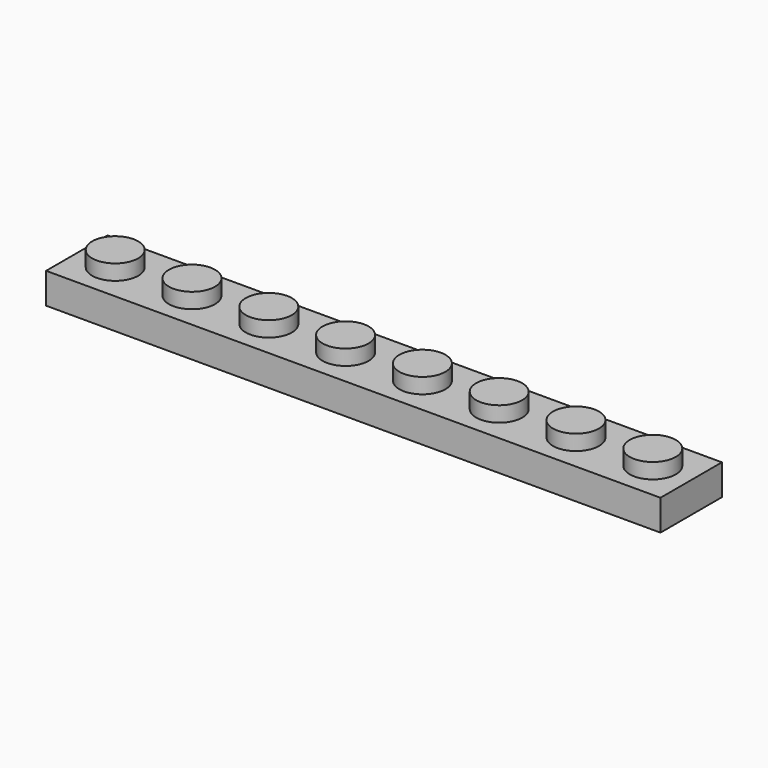
from build123d import *

# Parameters (mm, degrees)
F0_W     = 63.5
F0_H     = 7.9375
F0_R     = 2.38125
F1_DEPTH = 3.175
F2_DEPTH = 4.7625
F3_T     = -1.5875
F4_R     = 1.5875
F4_R_2   = 0.79375
F5_DEPTH = 1.5875


# Not quite as in the source:
# - a feature names something its author has since deleted; it is built from what else it names


with BuildPart() as f1:
    # F0 (on Top) → F1 (new body)
    with BuildSketch(Plane.XY):
        Rectangle(F0_W, F0_H)
        with Locations((-27.78125, 0)):
            Circle(F0_R, mode=Mode.SUBTRACT)
        with Locations((-19.84375, 0)):
            Circle(F0_R, mode=Mode.SUBTRACT)
        with Locations((-11.90625, 0)):
            Circle(F0_R, mode=Mode.SUBTRACT)
        with Locations((-3.96875, 0)):
            Circle(F0_R, mode=Mode.SUBTRACT)
        with Locations((3.96875, 0)):
            Circle(F0_R, mode=Mode.SUBTRACT)
        with Locations((11.90625, 0)):
            Circle(F0_R, mode=Mode.SUBTRACT)
        with Locations((19.84375, 0)):
            Circle(F0_R, mode=Mode.SUBTRACT)
        with Locations((27.78125, 0)):
            Circle(F0_R, mode=Mode.SUBTRACT)
    extrude(amount=F1_DEPTH)

    # F0 (on Top) → F2 (join)
    with BuildSketch(Plane.XY):
        with Locations((-27.78125, 0)):
            Circle(F0_R)
        with Locations((-11.90625, 0)):
            Circle(F0_R)
        with Locations((-19.84375, 0)):
            Circle(F0_R)
        with Locations((-3.96875, 0)):
            Circle(F0_R)
        with Locations((3.96875, 0)):
            Circle(F0_R)
        with Locations((11.90625, 0)):
            Circle(F0_R)
        with Locations((19.84375, 0)):
            Circle(F0_R)
        with Locations((27.78125, 0)):
            Circle(F0_R)
    extrude(amount=F2_DEPTH)

    # F3
    f3_openings = [f1.faces().sort_by_distance(p)[0] for p in [
        (0, 0, 0),
    ]]
    offset(amount=F3_T, openings=f3_openings, kind=Kind.INTERSECTION)

    # F4 (on face) → F5 (join)
    with BuildSketch(Plane(origin=(0, 0, 1.5875), x_dir=(1, 0, 0), z_dir=(0, 0, -1))):
        with Locations((-23.8125, 0)):
            Circle(F4_R)
        with Locations((-23.8125, 0)):
            Circle(F4_R_2, mode=Mode.SUBTRACT)
        with Locations((-15.875, 0)):
            Circle(F4_R)
        with Locations((-15.875, 0)):
            Circle(F4_R_2, mode=Mode.SUBTRACT)
        with Locations((-7.9375, 0)):
            Circle(F4_R)
        with Locations((-7.9375, 0)):
            Circle(F4_R_2, mode=Mode.SUBTRACT)
        Circle(F4_R)
        Circle(F4_R_2, mode=Mode.SUBTRACT)
        with Locations((7.9375, 0)):
            Circle(F4_R)
        with Locations((7.9375, 0)):
            Circle(F4_R_2, mode=Mode.SUBTRACT)
        with Locations((15.875, 0)):
            Circle(F4_R)
        with Locations((15.875, 0)):
            Circle(F4_R_2, mode=Mode.SUBTRACT)
        with Locations((23.8125, 0)):
            Circle(F4_R)
        with Locations((23.8125, 0)):
            Circle(F4_R_2, mode=Mode.SUBTRACT)
    extrude(amount=F5_DEPTH)


solid = f1.part
